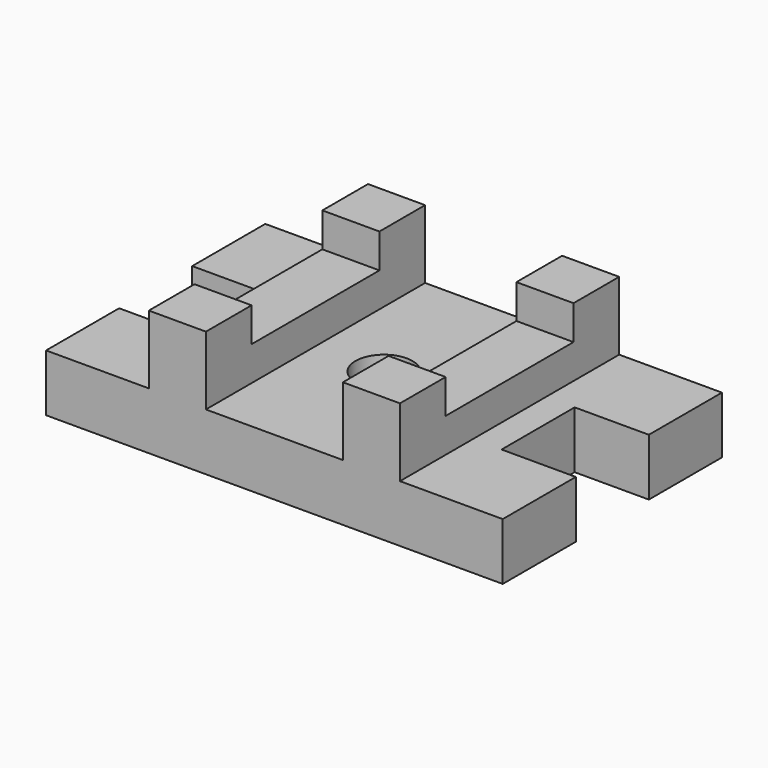
from build123d import *

# Parameters (mm, degrees)
F1_DEPTH = 31.75
F0_R     = 15.875
F0_W     = 31.75
F0_H     = 88.9
F2_DEPTH = 50.8
F0_H_2   = 31.75
F3_DEPTH = 69.85


# Not quite as in the source:
# - a feature names something its author has since deleted; it is built from what else it names


with BuildPart() as f1:
    # F0 (on Top) → F1 (new body)
    with BuildSketch(Plane.XY):
        Polygon((-69.85, 44.45), (-69.85, 76.2), (-127, 76.2), (-127, 25.4), (-85.725, 25.4), (-85.725, -25.4), (-127, -25.4), (-127, -76.2), (-69.85, -76.2), (-69.85, -44.45), align=None)
    extrude(amount=F1_DEPTH)



with BuildPart() as f1b:
    # F0 (on Top) → F1, piece 2 (new body)
    with BuildSketch(Plane.XY):
        Polygon((38.1, 44.45), (38.1, 76.2), (-38.1, 76.2), (-38.1, 44.45), (-38.1, -44.45), (-38.1, -76.2), (38.1, -76.2), (38.1, -44.45), align=None)
        Circle(F0_R, mode=Mode.SUBTRACT)
    extrude(amount=F1_DEPTH)


with BuildPart() as f1c:
    # F0 (on Top) → F1, piece 3 (new body)
    with BuildSketch(Plane.XY):
        Polygon((127, 76.2), (69.85, 76.2), (69.85, 44.45), (69.85, -44.45), (69.85, -76.2), (127, -76.2), (127, -25.4), (85.725, -25.4), (85.725, 25.4), (127, 25.4), align=None)
    extrude(amount=F1_DEPTH)


with BuildPart() as f1_1:
    add(f1.part)

    add(f1b.part)  # F2 merges F1b

    add(f1c.part)  # F2 merges F1c
    # F0 (on Top) → F2 (join)
    with BuildSketch(Plane.XY):
        with Locations((-53.975, 0)):
            Rectangle(F0_W, F0_H)
        with Locations((53.975, 0)):
            Rectangle(F0_W, F0_H)
    extrude(amount=F2_DEPTH)

    # F0 (on Top) → F3 (join)
    with BuildSketch(Plane.XY):
        with Locations((53.975, -60.325)):
            Rectangle(F0_W, F0_H_2)
        with Locations((-53.975, 60.325)):
            Rectangle(F0_W, F0_H_2)
        with Locations((-53.975, -60.325)):
            Rectangle(F0_W, F0_H_2)
        with Locations((53.975, 60.325)):
            Rectangle(F0_W, F0_H_2)
    extrude(amount=F3_DEPTH)


solid = f1_1.part
